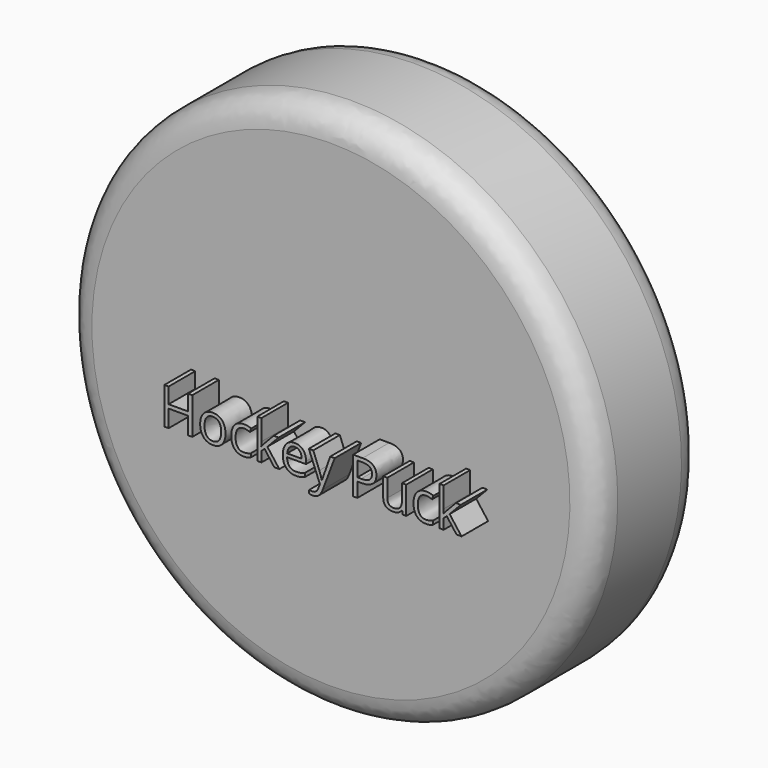
from build123d import *

# Parameters (mm, degrees)
F1_DEPTH     = 25.4
F2_R         = 5.08
F3_TEXT_SIZE = 9.8422059738
F4_DEPTH     = 6.35


# Not quite as in the source:
# - Text() gives the source's letters only with a copy of the font that has no kerning and outlines rounded to 1/6400 em; it was checked with that copy


with BuildPart() as f1:
    # F0 (on Front) → F1 (new body)
    with BuildSketch(Plane.XZ):
        with BuildLine():
            add(Edge.make_bspline(
                [(6.5287026737, 56.6721749642), (-81.2233431535, 63.1141042662), (-42.9261946648, -16.1023613053), (-4.6290461761, -95.3188268767), (44.8258511624, -22.5442906073), (94.280748501, 50.2302456622), (6.5287026737, 56.6721749642)],
                knots=[0, 0, 0, 2.0943951024, 2.0943951024, 4.1887902048, 4.1887902048, 6.2831853072, 6.2831853072, 6.2831853072], degree=2, weights=[1, 0.5, 1, 0.5, 1, 0.5, 1]))
        make_face()
    extrude(amount=F1_DEPTH)

    # F2
    f2_edges = [f1.edges().sort_by_distance(p)[0] for p in [
        (-0.909797, -25.4, -44.65516),
        (-0.909797, 0, -44.65516),
    ]]
    fillet(f2_edges, radius=F2_R)

    # F3 (on face) → F4 (join)
    with BuildSketch(Plane.XZ.offset(25.4)):
        with Locations((-24.9274633825, -2.1330467425)):
            Text('Hockey Puck', F3_TEXT_SIZE, font='Open Sans', text_align=(TextAlign.LEFT, TextAlign.BOTTOM))
    extrude(amount=F4_DEPTH)


solid = f1.part
